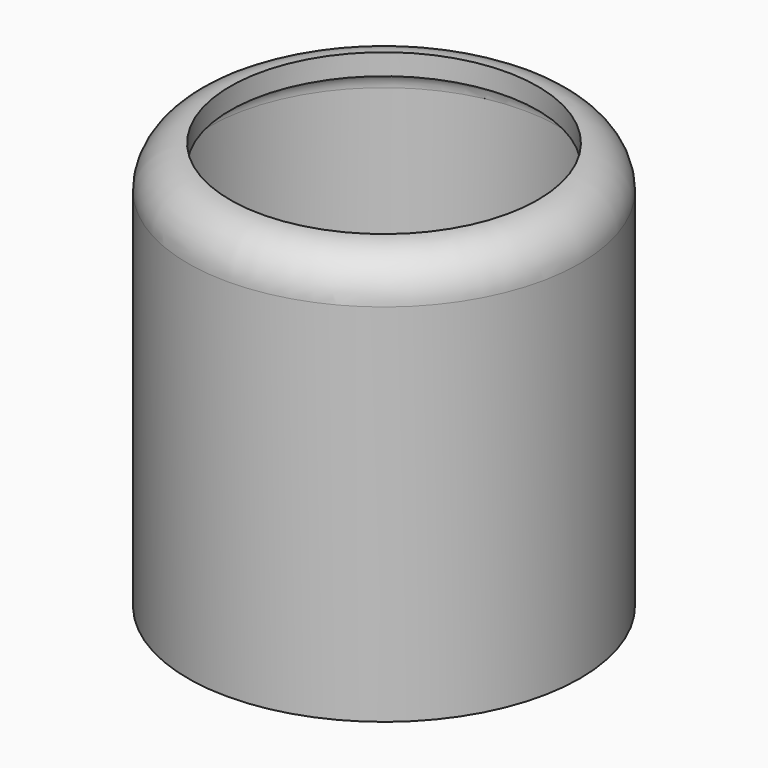
from build123d import *

# Parameters (mm, degrees)
F0_R     = 23.5821475326
F1_DEPTH = 49.022
F2_R     = 5.08
F3_T     = -2.54


# Not quite as in the source:
# - a shell that OpenCascade refuses in one call is made with other operations: the cavity is built on its own and cut out


with BuildPart() as f1:
    # F0 (on Top) → F1 (new body)
    with BuildSketch(Plane.XY):
        with Locations((-6.0959998518, 30.3276013583)):
            Circle(F0_R)
    extrude(amount=F1_DEPTH)

    # F2
    f2_edges = [f1.edges().sort_by_distance(p)[0] for p in [
        (-29.678147, 30.327601, 49.022),
    ]]
    fillet(f2_edges, radius=F2_R)

    # F3: a shell. OpenCascade refuses it in one call, so the cavity is built on its own and cut out:
    # the body offset inwards by the wall thickness, plus a prism from it out through each open face.
    f3_core = offset(f1.part, amount=F3_T, mode=Mode.PRIVATE)
    f3_exits = [f3_core.faces().sort_by_distance(p)[0] for p in [
        (-6.096, 30.327601, 46.482),
    ]]
    add(f3_core, mode=Mode.SUBTRACT)
    extrude(f3_exits, amount=-F3_T, mode=Mode.SUBTRACT)


solid = f1.part
